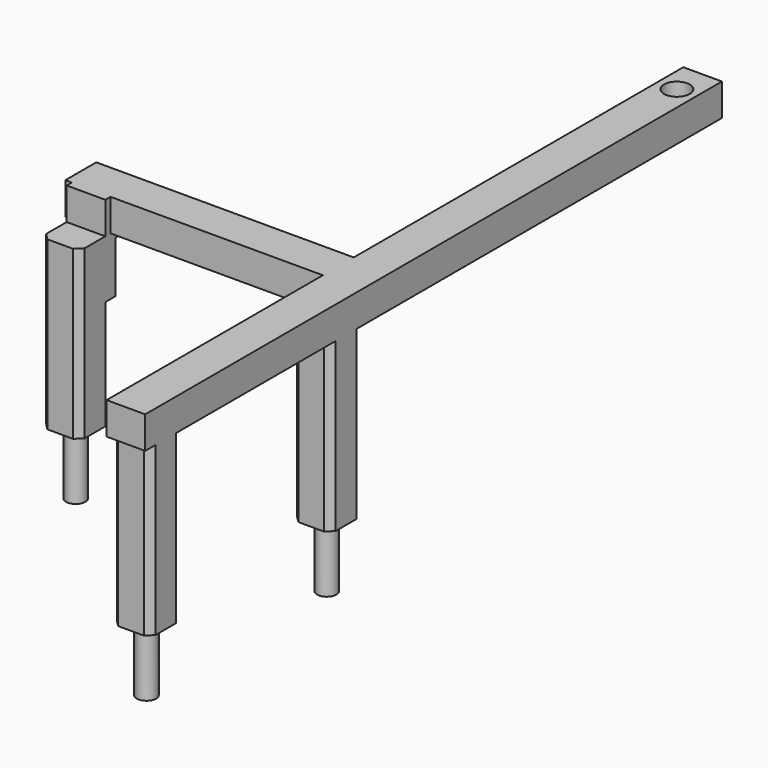
from build123d import *

# Parameters (mm, degrees)
F0_W      = 30
F0_H      = 25
F1_DEPTH  = 560
F2_W      = 30
F2_H      = 25
F3_DEPTH  = 200
F4_R      = 10
F5_DEPTH  = 25
F6_W      = 30
F6_H      = 30
F7_DEPTH  = 130
F8_SIZE   = 5
F9_R      = 7.5
F9_R_2    = 4
F10_DEPTH = 50
F12_R     = 7.5
F12_R_2   = 4
F13_DEPTH = 50
F14_W     = 30
F14_H     = 30
F15_DEPTH = 5
F16_W     = 30
F16_H     = 5
F17_DEPTH = 40
F18_W     = 30
F18_H     = 130
F19_DEPTH = 30
F20_SIZE  = 5
F21_R     = 7.5
F21_R_2   = 4
F22_DEPTH = 50
F23_W     = 30
F23_H     = 5
F24_DEPTH = 25


# Not quite as in the source:
# - two fillets or chamfers of one size are made in one step


with BuildPart() as f1:
    # F0 (on Front) → F1 (new body)
    with BuildSketch(Plane.XZ):
        Rectangle(F0_W, F0_H)
    extrude(amount=F1_DEPTH)

    # F2 (on face) → F3 (join)
    with BuildSketch(Plane(origin=(-15, 0, 0), x_dir=(0, -1, 0), z_dir=(-1, 0, 0))):
        with Locations((335, 0)):
            Rectangle(F2_W, F2_H)
    extrude(amount=F3_DEPTH)

    # F4 (on face) → F5 (cut)
    with BuildSketch(Plane.XY.offset(12.5)):
        with Locations((0, -25)):
            Circle(F4_R)
    extrude(amount=-F5_DEPTH, mode=Mode.SUBTRACT)

    # F6 (on face) → F7 (join)
    with BuildSketch(Plane(origin=(0, 0, -12.5), x_dir=(1, 0, 0), z_dir=(0, 0, -1))):
        with Locations((0, 540)):
            Rectangle(F6_W, F6_H)
        with Locations((0, 365)):
            Rectangle(F6_W, F6_H)
    extrude(amount=F7_DEPTH)

    # F8
    f8_edges = [f1.edges().sort_by_distance(p)[0] for p in [
        (-15, -555, -77.5),
        (15, -555, -77.5),
        (15, -525, -77.5),
        (-15, -525, -77.5),
        (15, -350, -77.5),
        (15, -380, -77.5),
        (-15, -350, -77.5),
        (-15, -380, -77.5),
    ]]
    chamfer(f8_edges, length=F8_SIZE)

    # F9 (on face) → F10 (join)
    with BuildSketch(Plane(origin=(0, 0, -142.5), x_dir=(1, 0, 0), z_dir=(0, 0, -1))):
        with Locations((0, 540)):
            Circle(F9_R)
        with Locations((0, 540)):
            Circle(F9_R_2, mode=Mode.SUBTRACT)
    extrude(amount=F10_DEPTH)

    # F12 (on face) → F13 (join)
    with BuildSketch(Plane(origin=(0, 0, -142.5), x_dir=(1, 0, 0), z_dir=(0, 0, -1))):
        with Locations((0, 365)):
            Circle(F12_R)
        with Locations((0, 365)):
            Circle(F12_R_2, mode=Mode.SUBTRACT)
    extrude(amount=F13_DEPTH)

    # F14 (on face) → F15 (join)
    with BuildSketch(Plane(origin=(0, 0, -12.5), x_dir=(1, 0, 0), z_dir=(0, 0, -1))):
        with Locations((-195, 335)):
            Rectangle(F14_W, F14_H)
    extrude(amount=F15_DEPTH)

    # F16 (on face) → F17 (join)
    with BuildSketch(Plane(origin=(0, 0, -17.5), x_dir=(1, 0, 0), z_dir=(0, 0, -1))):
        with Locations((-195, 347.5)):
            Rectangle(F16_W, F16_H)
    extrude(amount=F17_DEPTH)

    # F18 (on face) → F19 (join)
    with BuildSketch(Plane.XZ.offset(350)):
        with Locations((-195, -77.5)):
            Rectangle(F18_W, F18_H)
    extrude(amount=F19_DEPTH)

    # F20
    f20_edges = [f1.edges().sort_by_distance(p)[0] for p in [
        (-210, -380, -77.5),
        (-180, -380, -77.5),
        (-180, -350, -100),
        (-210, -350, -100),
    ]]
    chamfer(f20_edges, length=F20_SIZE)

    # F21 (on face) → F22 (join)
    with BuildSketch(Plane(origin=(0, 0, -142.5), x_dir=(1, 0, 0), z_dir=(0, 0, -1))):
        with Locations((-195, 365)):
            Circle(F21_R)
        with Locations((-195, 365)):
            Circle(F21_R_2, mode=Mode.SUBTRACT)
    extrude(amount=F22_DEPTH)

    # F23 (on face) → F24 (join)
    with BuildSketch(Plane.XY.offset(-12.5)):
        with Locations((-195, -352.5)):
            Rectangle(F23_W, F23_H)
    extrude(amount=F24_DEPTH)


solid = f1.part
